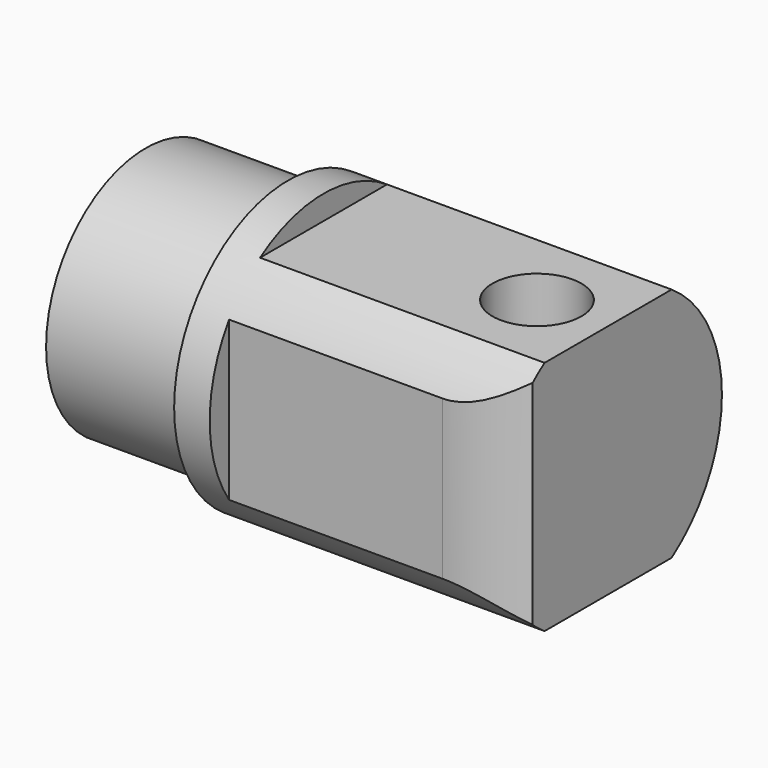
from build123d import *

# Parameters (mm, degrees)
F0_R     = 12.7
F1_DEPTH = 28.575
F2_R     = 11.1125
F3_DEPTH = 12.7
F5_DEPTH = 25.4
F6_R     = 3.96875
F7_DEPTH = 23.242
F9_DEPTH = 23.242


with BuildPart() as f1:
    # F0 (on Right) → F1 (new body)
    with BuildSketch(Plane.YZ):
        Circle(F0_R)
    extrude(amount=F1_DEPTH)

    # F2 (on face) → F3 (join)
    with BuildSketch(Plane(origin=(0, 0, 0), x_dir=(0, -1, 0), z_dir=(-1, 0, 0))):
        Circle(F2_R)
    extrude(amount=F3_DEPTH)

    # F4 (on face) → F5 (cut)
    with BuildSketch(Plane.YZ.offset(28.575)):
        with BuildLine():
            Line((-10.541, 7.0835950618), (-10.541, 10.541))
            Line((-10.541, 10.541), (-7.0835950618, 10.541))
            ThreePointArc((-7.0835950618, 10.541), (0, 12.7), (7.0835950618, 10.541))
            Line((7.0835950618, 10.541), (14.6175222471, 10.541))
            Line((14.6175222471, 10.541), (14.6175222471, 13.3875589818))
            Line((14.6175222471, 13.3875589818), (-14.6175222471, 13.3875589818))
            Line((-14.6175222471, 13.3875589818), (-14.6175222471, -13.3875589818))
            Line((-14.6175222471, -13.3875589818), (14.6175222471, -13.3875589818))
            Line((14.6175222471, -13.3875589818), (14.6175222471, -10.541))
            Line((14.6175222471, -10.541), (7.0835950618, -10.541))
            ThreePointArc((7.0835950618, -10.541), (0, -12.7), (-7.0835950618, -10.541))
            Line((-7.0835950618, -10.541), (-10.541, -10.541))
            Line((-10.541, -10.541), (-10.541, -7.0835950618))
            ThreePointArc((-10.541, -7.0835950618), (-12.7, 0), (-10.541, 7.0835950618))
        make_face()
        with BuildLine():
            ThreePointArc((7.0835950618, 10.541), (0, 12.7), (-7.0835950618, 10.541))
            Line((-7.0835950618, 10.541), (7.0835950618, 10.541))
        make_face()
        with BuildLine():
            Line((-10.541, -7.0835950618), (-10.541, 7.0835950618))
            ThreePointArc((-10.541, 7.0835950618), (-12.7, 0), (-10.541, -7.0835950618))
        make_face()
        with BuildLine():
            Line((7.0835950618, -10.541), (-7.0835950618, -10.541))
            ThreePointArc((-7.0835950618, -10.541), (0, -12.7), (7.0835950618, -10.541))
        make_face()
    extrude(amount=-F5_DEPTH, mode=Mode.SUBTRACT)

    # F6 (on face) → F7 (cut, through all)
    with BuildSketch(Plane.XY.offset(10.541)):
        with Locations((22.225, 0)):
            Circle(F6_R)
    extrude(amount=-F7_DEPTH, mode=Mode.SUBTRACT)

    # F8 (on face) → F9 (cut, through all)
    with BuildSketch(Plane.XY.offset(10.541)):
        with BuildLine():
            ThreePointArc((32.766, 0), (29.6786125805, -7.4536125805), (22.225, -10.541))
            Line((22.225, -10.541), (22.225, -14.2959095994))
            ThreePointArc((22.225, -14.2959095994), (32.333734621, -10.108734621), (36.5209095994, 0))
            Line((36.5209095994, 0), (32.766, 0))
        make_face()
    extrude(amount=-F9_DEPTH, mode=Mode.SUBTRACT)


solid = f1.part
